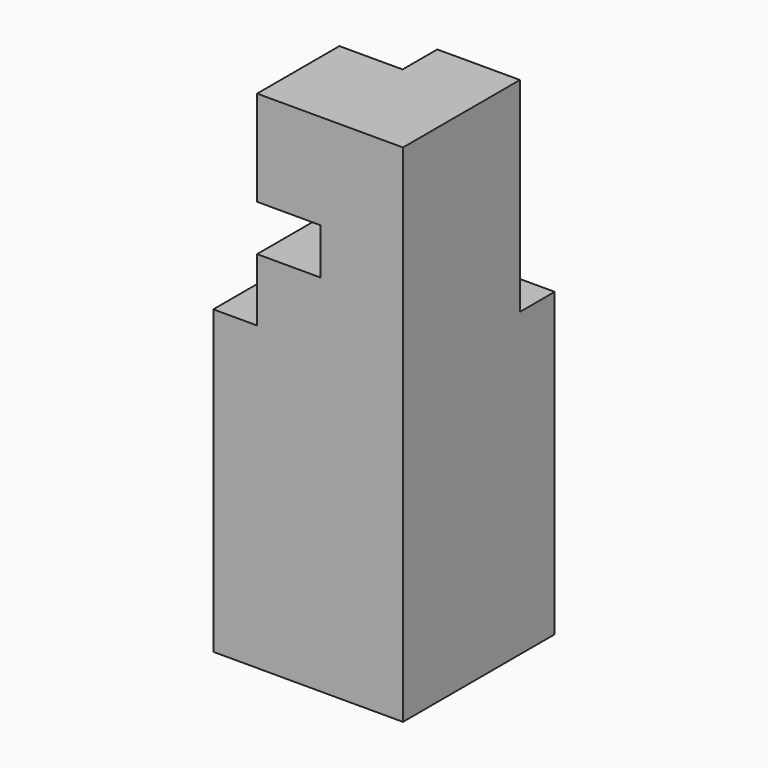
from build123d import *

# Parameters (mm, degrees)
F0_W     = 19.05
F0_H     = 19.05
F1_DEPTH = 50.8
F2_W     = 4.3630654678
F2_H     = 20.508804819
F3_DEPTH = 25.4
F4_W     = 4.3975393042
F4_H     = 20.508804819
F5_DEPTH = 25.4
F6_W     = 4.3544375803
F6_H     = 20.508804819
F7_DEPTH = 6.35
F8_W     = 6.35
F8_H     = 4.6250596642
F9_DEPTH = 25.4


# Not quite as in the source:
# - a feature names something its author has since deleted; it is built from what else it names


with BuildPart() as f1:
    # F0 (on Top) → F1 (new body)
    with BuildSketch(Plane.XY):
        Rectangle(F0_W, F0_H)
    extrude(amount=F1_DEPTH)

    # F2 (on face) → F3 (cut)
    with BuildSketch(Plane.YZ.offset(9.525)):
        with Locations((7.3434672661, 40.5455975905)):
            Rectangle(F2_W, F2_H)
    extrude(amount=-F3_DEPTH, mode=Mode.SUBTRACT)

    # F4 (on face) → F5 (cut)
    with BuildSketch(Plane(origin=(0, 5.1619345322, 0), x_dir=(-1, 0, 0), z_dir=(0, 1, 0))):
        with Locations((7.3262303479, 40.5455975905)):
            Rectangle(F4_W, F4_H)
    extrude(amount=-F5_DEPTH, mode=Mode.SUBTRACT)

    # F6 (on face) → F7 (cut)
    with BuildSketch(Plane(origin=(-5.1274606958, 0, 0), x_dir=(0, -1, 0), z_dir=(-1, 0, 0))):
        with Locations((-2.9847157421, 40.5455975905)):
            Rectangle(F6_W, F6_H)
    extrude(amount=-F7_DEPTH, mode=Mode.SUBTRACT)

    # F8 (on face) → F9 (cut)
    with BuildSketch(Plane(origin=(0, 0.8074969519, 0), x_dir=(-1, 0, 0), z_dir=(0, 1, 0))):
        with Locations((1.9524606958, 38.9165244997)):
            Rectangle(F8_W, F8_H)
    extrude(amount=-F9_DEPTH, mode=Mode.SUBTRACT)


solid = f1.part
